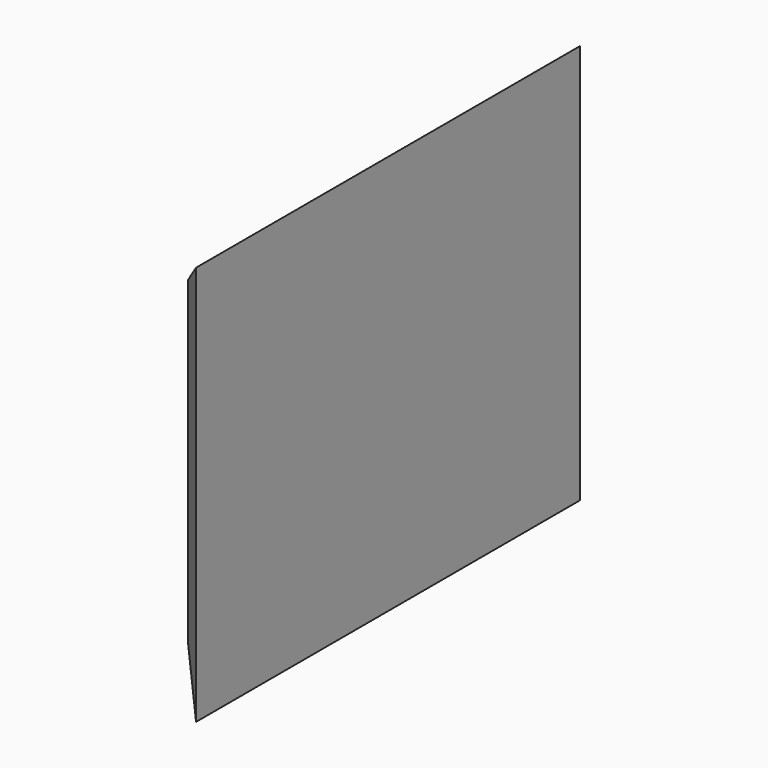
from build123d import *

# Parameters (mm, degrees)
F0_W     = 300
F0_H     = 250
F1_DEPTH = 25
F2_SIZE  = 24.99999


# Not quite as in the source:
# - a fillet or chamfer is up to 0.001 mm smaller than in the source, because OpenCascade refuses the exact size


with BuildPart() as f1:
    # F0 (on Right) → F1 (new body)
    with BuildSketch(Plane.YZ):
        Rectangle(F0_W, F0_H)
    extrude(amount=-F1_DEPTH)

    # F2 (size 25 in the source; OpenCascade refuses exactly that, so slightly less here)
    f2_edges = [f1.edges().sort_by_distance(p)[0] for p in [
        (-25, 0, 125),
        (-25, -150, 0),
        (-25, 0, -125),
        (-25, 150, 0),
    ]]
    chamfer(f2_edges, length=F2_SIZE)


solid = f1.part
